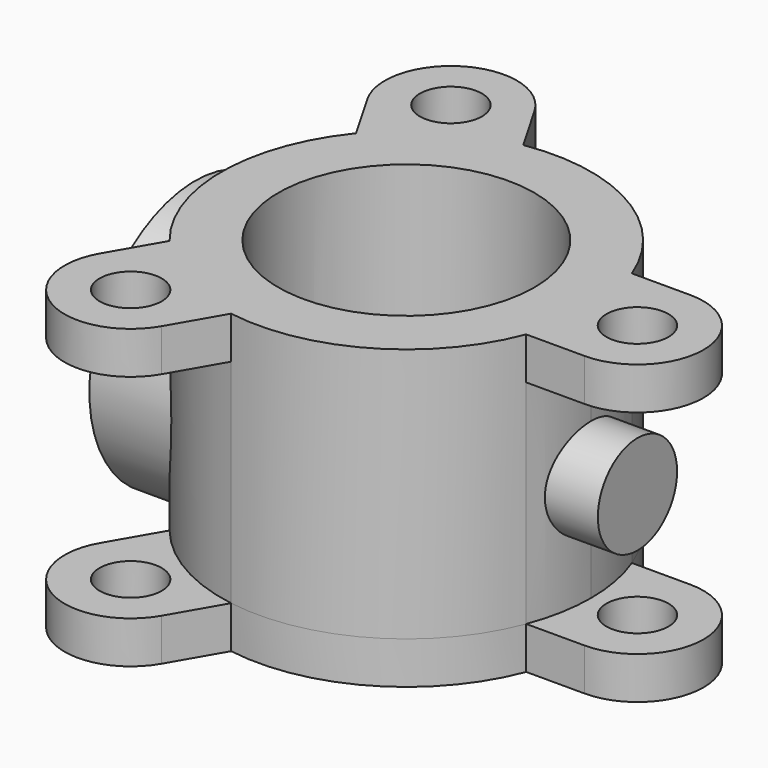
from build123d import *

# Parameters (mm, degrees)
F0_R            = 97
F0_R_2          = 23.5
F1_DEPTH        = 32
F2_COUNT        = 3
F2_ANGLE        = 240
F3_R            = 97
F4_DEPTH        = 161
F5_R            = 23.5
F5_R_2          = 97
F6_DEPTH        = 32
F8_R            = 100
F12_D           = 20.3
F12_DEPTH       = 15
F12_TIP         = 6.098735
F14_R           = 37.5
F16_D           = 56.2
F16_DEPTH       = 310
F16_CBORE_D     = 100
F16_CBORE_DEPTH = 25
F16_TIP         = 16.884183


with BuildPart() as f1:
    # F0 (on Top) → F1 (new body)
    with BuildSketch(Plane.XY):
        with BuildLine():
            Line((175, 50), (130.766968, 50))
            ThreePointArc((130.766968, 50), (-140, 0), (130.766968, -50))
            Line((130.766968, -50), (175, -50))
            ThreePointArc((175, -50), (225, 0), (175, 50))
        make_face()
        Circle(F0_R, mode=Mode.SUBTRACT)
        with Locations((175, 0)):
            Circle(F0_R_2, mode=Mode.SUBTRACT)
    extrude(amount=F1_DEPTH)

    # F2: F1 ×3 about axis
    f2_axis = Axis((0, 0, 32), (0, 0, 1))


with BuildPart() as f1_1:
    add(f1.part)
    for i in range(1, F2_COUNT):
        add(f1.part.rotate(f2_axis, i * F2_ANGLE / (F2_COUNT - 1)))

    # F3 (on face) → F4 (join)
    with BuildSketch(Plane.XY.offset(32)):
        with BuildLine():
            ThreePointArc((130.766968, -50), (137.672393, -25.422671), (140, 0))
            ThreePointArc((140, 0), (137.672393, 25.422671), (130.766968, 50))
            ThreePointArc((130.766968, 50), (70, 121.243557), (-22.082214, 138.247517))
            ThreePointArc((-22.082214, 138.247517), (-70, 121.243557), (-108.684754, 88.247517))
            ThreePointArc((-108.684754, 88.247517), (-140, 0), (-108.684754, -88.247517))
            ThreePointArc((-108.684754, -88.247517), (-70, -121.243557), (-22.082214, -138.247517))
            ThreePointArc((-22.082214, -138.247517), (70, -121.243557), (130.766968, -50))
        make_face()
        Circle(F3_R, mode=Mode.SUBTRACT)
    extrude(amount=F4_DEPTH)

    # F5 (on face) → F6 (join)
    with BuildSketch(Plane.XY.offset(193)):
        with BuildLine():
            Line((130.766968, -50), (175, -50))
            ThreePointArc((175, -50), (225, 0), (175, 50))
            Line((175, 50), (130.766968, 50))
            ThreePointArc((130.766968, 50), (70, 121.243557), (-22.082214, 138.247517))
            Line((-22.082214, 138.247517), (-44.19873, 176.554446))
            ThreePointArc((-44.19873, 176.554446), (-112.5, 194.855716), (-130.80127, 126.554446))
            Line((-130.80127, 126.554446), (-108.684754, 88.247517))
            ThreePointArc((-108.684754, 88.247517), (-140, 0), (-108.684754, -88.247517))
            Line((-108.684754, -88.247517), (-130.80127, -126.554446))
            ThreePointArc((-130.80127, -126.554446), (-112.5, -194.855716), (-44.19873, -176.554446))
            Line((-44.19873, -176.554446), (-22.082214, -138.247517))
            ThreePointArc((-22.082214, -138.247517), (70, -121.243557), (130.766968, -50))
        make_face()
        with Locations((-87.5, -151.554446)):
            Circle(F5_R, mode=Mode.SUBTRACT)
        Circle(F5_R_2, mode=Mode.SUBTRACT)
        with Locations((175, 0)):
            Circle(F5_R, mode=Mode.SUBTRACT)
        with Locations((-87.5, 151.554446)):
            Circle(F5_R, mode=Mode.SUBTRACT)
    extrude(amount=F6_DEPTH)

    # F8 (on offset) → F9 (join, up to the next surface of F1)
    with BuildSketch(Plane.YZ.offset(-160)):
        with Locations((0, 112.5)):
            Circle(F8_R)
    extrude(until=Until.NEXT)

    # F12
    with Locations(Plane(origin=(-160, 0, 0), x_dir=(0, -1, 0), z_dir=(-1, 0, 0))):
        with Locations((0, 187.5), (-64.951905, 75), (64.951905, 75)):
            Hole(F12_D / 2, depth=F12_DEPTH)
            with Locations((0, 0, -(F12_DEPTH + F12_TIP / 2))):  # 118° drill point
                Cone(0, F12_D / 2, F12_TIP, mode=Mode.SUBTRACT)

    # F14 (on offset) → F15 (join, up to the next surface of F1)
    with BuildSketch(Plane.YZ.offset(175)):
        with Locations((0, 112.5)):
            Circle(F14_R)
    extrude(until=Until.NEXT, dir=(-1, 0, 0))

    # F16
    with Locations(Plane(origin=(-160, 0, 0), x_dir=(0, -1, 0), z_dir=(-1, 0, 0))):
        with Locations((0, 112.5)):
            CounterBoreHole(F16_D / 2, F16_CBORE_D / 2, F16_CBORE_DEPTH, depth=F16_DEPTH)
            with Locations((0, 0, -(F16_DEPTH + F16_TIP / 2))):  # 118° drill point
                Cone(0, F16_D / 2, F16_TIP, mode=Mode.SUBTRACT)


solid = f1_1.part
